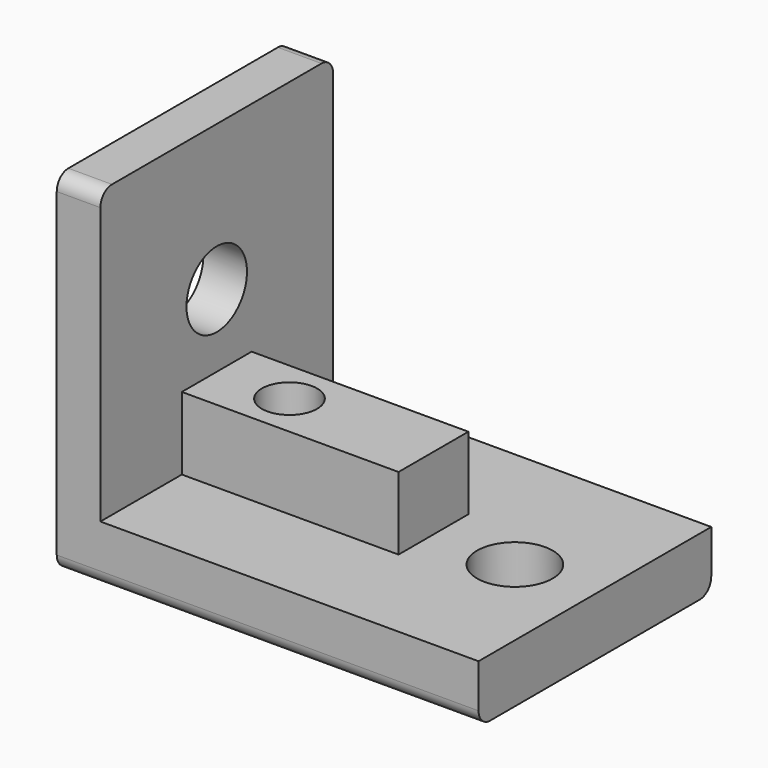
from build123d import *

# Parameters (mm, degrees)
F0_W      = 26
F0_H      = 20
F1_DEPTH  = 4
F2_W      = 26
F2_H      = 6
F3_DEPTH  = 5
F4_R      = 1.9
F5_DEPTH  = 25
F6_W      = 11.2
F6_H      = 6
F7_DEPTH  = 5
F8_R      = 2.6
F9_DEPTH  = 4
F10_R     = 2.6
F11_DEPTH = 3
F12_R     = 1


# Not quite as in the source:
# - a fillet or chamfer that OpenCascade refuses, or shapes differently, is made with other operations: its cross-section is extruded or revolved along the edge and cut away or added
# - a feature names something its author has since deleted; it is built from what else it names


with BuildPart() as f1:
    # F0 (on Top) → F1 (new body)
    with BuildSketch(Plane.XY):
        with Locations((13, 0)):
            Rectangle(F0_W, F0_H)
    extrude(amount=F1_DEPTH)

    # F2 (on face) → F3 (join)
    with BuildSketch(Plane.XY.offset(4)):
        with Locations((13, 0)):
            Rectangle(F2_W, F2_H)
    extrude(amount=F3_DEPTH)

    # F4 (on face) → F5 (cut)
    with BuildSketch(Plane.XY.offset(9)):
        with Locations((5, 0)):
            Circle(F4_R)
    extrude(amount=-F5_DEPTH, mode=Mode.SUBTRACT)

    # F6 (on face) → F7 (cut, through all)
    with BuildSketch(Plane.XY.offset(9)):
        with Locations((20.5, 0)):
            Rectangle(F6_W, F6_H)
    extrude(amount=-F7_DEPTH, mode=Mode.SUBTRACT)

    # F8 (on face) → F9 (cut, through all)
    with BuildSketch(Plane.XY.offset(4)):
        with Locations((20.5, 0)):
            Circle(F8_R)
    extrude(amount=-F9_DEPTH, mode=Mode.SUBTRACT)

    # F10 (on face) → F11 (join)
    with BuildSketch(Plane(origin=(0, 0, 0), x_dir=(0, -1, 0), z_dir=(-1, 0, 0))):
        Polygon((-10, 24), (-10, 4), (-3, 4), (-3, 9), (3, 9), (3, 4), (10, 4), (10, 24), align=None)
        with Locations((0, 14)):
            Circle(F10_R, mode=Mode.SUBTRACT)
        Polygon((-10, 4), (-10, 0), (10, 0), (10, 4), (3, 4), (3, 9), (-3, 9), (-3, 4), align=None)
    extrude(amount=F11_DEPTH)

    # F12
    f12_edges = [f1.edges().sort_by_distance(p)[0] for p in [
        (-1.5, -10, 24),
        (-1.5, 10, 24),
        (11.5, -10, 0),
        (11.5, 10, 0),
    ]]
    fillet(f12_edges, radius=F12_R)

    # F13: chamfer of 0.5 x 0.2886751346 on 1 edges, made by hand

    # F13_s1 → F13_t2 (revolve, cut)
    with BuildSketch(Plane.XZ):
        Polygon((7.1886751346, 0), (6.9, 0.5), (6.9, 0), align=None)
    revolve(axis=Axis((5, 0, 0), (0, 0, 1)), mode=Mode.SUBTRACT)


solid = f1.part
